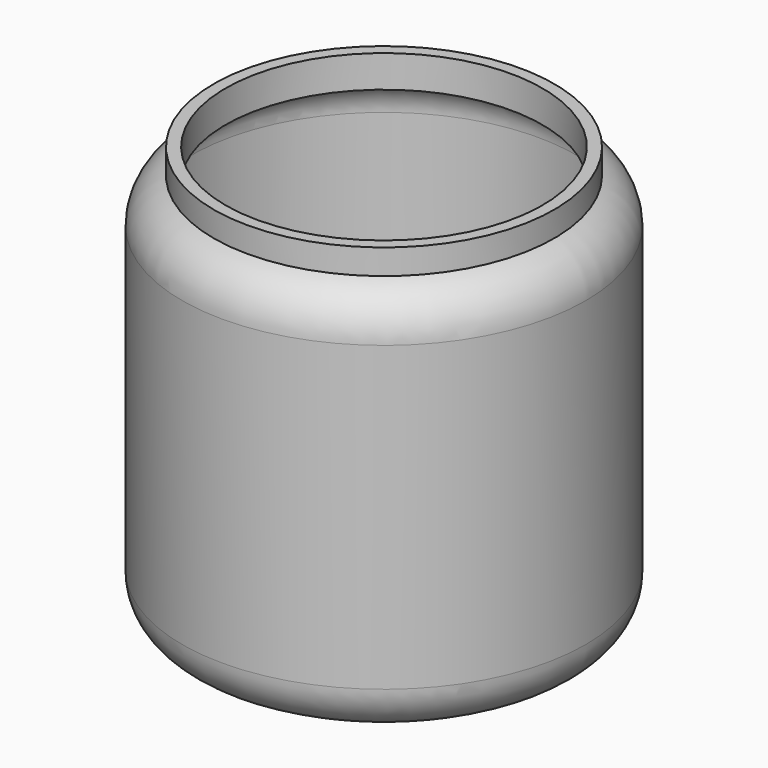
from build123d import *

# Parameters (mm, degrees)
F0_R     = 101.6
F0_R_2   = 96.8375
F1_DEPTH = 152.4
F4_DEPTH = 12.7


with BuildPart() as f1:
    # F0 (on Top) → F1 (new body)
    with BuildSketch(Plane.XY):
        Circle(F0_R)
        Circle(F0_R_2, mode=Mode.SUBTRACT)
    extrude(amount=F1_DEPTH)

    # F2 (on Right) → F3 (revolve)
    with BuildSketch(Plane.YZ):
        with BuildLine():
            Line((-101.6, 152.4), (-96.8375, 152.4))
            ThreePointArc((-96.8375, 152.4), (-93.8204640896, 162.6881758587), (-85.725, 169.717580482))
            ThreePointArc((-85.725, 169.717580482), (-82.8148388415, 170.774666369), (-79.771875, 171.3463652414))
            Line((-79.771875, 171.3463652414), (-79.771875, 174.8506403027))
            Line((-79.771875, 174.8506403027), (-81.75625, 174.8506403027))
            Line((-81.75625, 174.8506403027), (-85.725, 174.8506403027))
            ThreePointArc((-85.725, 174.8506403027), (-97.2303248333, 166.1481532851), (-101.6, 152.4))
        make_face()
    revolve(axis=Axis((0, 0, 76.2), (0, 0, 1)))

    # F4 (add): a face of the model
    f4_faces = [f1.faces().sort_by_distance(p)[0] for p in [
        (0, 82.1965441527, 174.8506403027),
    ]]
    extrude(f4_faces, amount=F4_DEPTH)

    # F5 (on Right) → F6 (revolve)
    with BuildSketch(Plane.YZ):
        with BuildLine():
            Line((0, -22.4506403027), (0, -19.05))
            Line((0, -19.05), (-77.7875, -19.05))
            ThreePointArc((-77.7875, -19.05), (-81.8496787146, -18.6118565461), (-85.725, -17.317580482))
            ThreePointArc((-85.725, -17.317580482), (-93.8204640896, -10.2881758587), (-96.8375, 0))
            Line((-96.8375, 0), (-101.6, 0))
            ThreePointArc((-101.6, 0), (-97.2303248333, -13.7481532851), (-85.725, -22.4506403027))
            Line((-85.725, -22.4506403027), (-77.7875, -22.4506403027))
            Line((-77.7875, -22.4506403027), (0, -22.4506403027))
        make_face()
    revolve(axis=Axis((0, 0, -11.2253201513), (0, 0, 1)))


solid = f1.part
